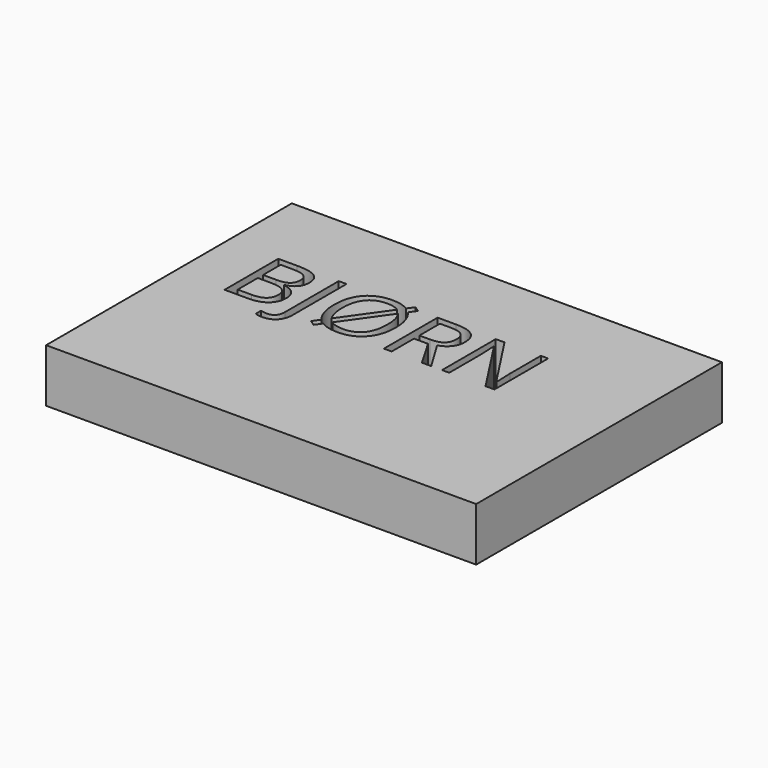
from build123d import *

# Parameters (mm, degrees)
F0_W         = 70
F0_H         = 50
F1_DEPTH     = 8.6848903447
F2_TEXT_SIZE = 15.3087855627
F3_DEPTH     = 25


# Not quite as in the source:
# - Text() gives the source's letters only with a copy of the font that has no kerning and outlines rounded to 1/6400 em; it was checked with that copy


with BuildPart() as f1:
    # F0 (on Top) → F1 (new body)
    with BuildSketch(Plane.XY):
        with Locations((42.4259601241, 38.3795835078)):
            Rectangle(F0_W, F0_H)
    extrude(amount=F1_DEPTH)

    # F2 (on face) → F3 (cut)
    with BuildSketch(Plane.XY.offset(8.6848903447)):
        with Locations((14.1095267609, 39.4583158195)):
            Text('BJØRN', F2_TEXT_SIZE, font='Open Sans', text_align=(TextAlign.LEFT, TextAlign.BOTTOM))
    extrude(amount=-F3_DEPTH, mode=Mode.SUBTRACT)


solid = f1.part
